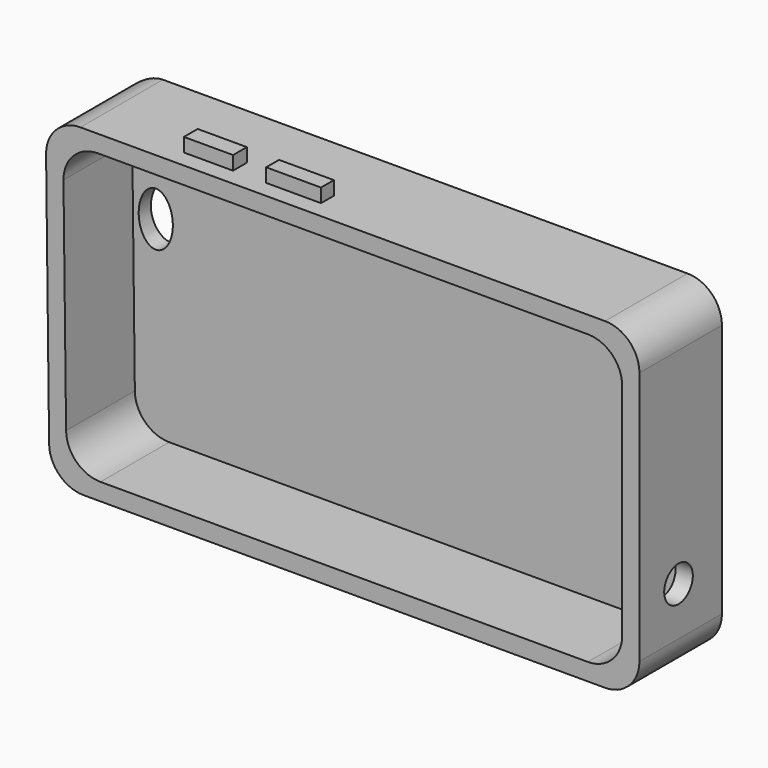
from build123d import *

# Parameters (mm, degrees)
F1_DEPTH    = 12.7
F2_T        = -2.54
F3_R        = 2.5336521523
F4_DEPTH    = 25.4
F5_W        = 12.6487519592
F5_H        = 3.011607565
F6_DEPTH    = 2.032
F7_T1_DEPTH = 51.1041796342
F7_T3_DEPTH = 73.1048124282
F7_T5_DEPTH = 50.4994199847
F7_T7_DEPTH = 50.8
F8_W        = 7.2596892715
F8_H        = 2.5458435994
F8_W_2      = 8.1038391218
F8_H_2      = 2.3770136759
F9_DEPTH    = 2.032
F11_DEPTH   = 5.334
F12_DEPTH   = 10.16
F13_R       = 5.08
F14_R       = 2.6429379381
F15_DEPTH   = 25.4


# Not quite as in the source:
# - a fillet or chamfer that OpenCascade refuses, or shapes differently, is made with other operations: its cross-section is extruded or revolved along the edge and cut away or added


with BuildPart() as f1:
    # F0 (on Front) → F1 (new body, symmetric)
    with BuildSketch(Plane.XZ):
        Polygon((37.1957607567, 37.33773157), (-50.5407974124, 37.33773157), (-49.9729253352, -10.3637007996), (37.1957607567, -10.3637007996), align=None)
    extrude(amount=F1_DEPTH, both=True)

    # F2
    f2_openings = [f1.faces().sort_by_distance(p)[0] for p in [
        (-6.530704, -12.7, 13.512828),
    ]]
    offset(amount=F2_T, openings=f2_openings)

    # F3 (on face) → F4 (cut)
    with BuildSketch(Plane.XZ.offset(-10.16)):
        with Locations((-44.7698123753, 30.0145167857)):
            Circle(F3_R)
    extrude(amount=-F4_DEPTH, mode=Mode.SUBTRACT)

    # F5 (on face) → F6 (join)
    with BuildSketch(Plane(origin=(0, 0, -10.3637007996), x_dir=(1, 0, 0), z_dir=(0, 0, -1))):
        with Locations((-34.2319430783, -6.4247637056)):
            Rectangle(F5_W, F5_H)
    extrude(amount=F6_DEPTH)

    # F7: fillet of radius 5.08 on 5 edges, made by hand

    # F7_s2 → F7_t1 (cut)
    with BuildSketch(Plane.XZ.offset(-25.5520898171)):
        with BuildLine():
            ThreePointArc((-50.4796015492, 32.19725989), (-49.0133806513, 35.8283900433), (-45.3999614856, 37.33773157))
            Line((-45.3999614856, 37.33773157), (-50.5407974124, 37.33773157))
            Line((-50.5407974124, 37.33773157), (-50.4796015492, 32.19725989))
        make_face()
    extrude(amount=F7_T1_DEPTH, mode=Mode.SUBTRACT)

    # F7_s4 → F7_t3 (cut)
    with BuildSketch(Plane(origin=(-0.602773104, 0, 50.6331295472), x_dir=(0, 1, 0), z_dir=(0.011903874, 0, -0.9999291464))):
        with BuildLine():
            ThreePointArc((12.7, -45.0127527613), (11.2121024484, -48.6048552097), (7.62, -50.0927527613))
            Line((7.62, -50.0927527613), (12.7, -50.0927527613))
            Line((12.7, -50.0927527613), (12.7, -45.0127527613))
        make_face()
    extrude(amount=F7_T3_DEPTH, mode=Mode.SUBTRACT)

    # F7_s6 → F7_t5 (cut)
    with BuildSketch(Plane.XZ.offset(-25.2497099923)):
        with BuildLine():
            ThreePointArc((-44.9530413382, -10.3637007996), (-48.5236998115, -8.8971199654), (-50.0326814019, -5.3441724797))
            Line((-50.0326814019, -5.3441724797), (-49.9729253352, -10.3637007996))
            Line((-49.9729253352, -10.3637007996), (-44.9530413382, -10.3637007996))
        make_face()
    extrude(amount=F7_T5_DEPTH, mode=Mode.SUBTRACT)

    # F7_s8 → F7_t7 (cut)
    with BuildSketch(Plane.XZ.offset(-25.4)):
        with BuildLine():
            ThreePointArc((32.1157607567, -10.3637007996), (35.7078632052, -8.8758032481), (37.1957607567, -5.2837007996))
            Line((37.1957607567, -5.2837007996), (37.1957607567, -10.3637007996))
            Line((37.1957607567, -10.3637007996), (32.1157607567, -10.3637007996))
        make_face()
        with BuildLine():
            ThreePointArc((37.1957607567, 32.25773157), (35.7078632052, 35.8498340184), (32.1157607567, 37.33773157))
            Line((32.1157607567, 37.33773157), (37.1957607567, 37.33773157))
            Line((37.1957607567, 37.33773157), (37.1957607567, 32.25773157))
        make_face()
    extrude(amount=F7_T7_DEPTH, mode=Mode.SUBTRACT)

    # F8 (on face) → F9 (join)
    with BuildSketch(Plane.XY.offset(37.33773157)):
        with Locations((-28.5155698657, 1.2729217997)):
            Rectangle(F8_W, F8_H)
        with Locations((-15.9377348609, 1.1885068379)):
            Rectangle(F8_W_2, F8_H_2)
    extrude(amount=F9_DEPTH)

    # F10 (on face) → F11 (cut)
    with BuildSketch(Plane.XZ.offset(-10.16)):
        with BuildLine():
            add(Edge.make_bspline(
                [(-44.4320701063, 24.525936693), (-48.8002594528, 24.525936693), (-46.6161647795, 18.5632575303), (-44.4320701063, 12.6005783677), (-42.247975433, 18.5632575303), (-40.0638807598, 24.525936693), (-44.4320701063, 24.525936693)],
                knots=[0, 0, 0, 2.0943951024, 2.0943951024, 4.1887902048, 4.1887902048, 6.2831853072, 6.2831853072, 6.2831853072], degree=2, weights=[1, 0.5, 1, 0.5, 1, 0.5, 1]))
        make_face()
    extrude(amount=-F11_DEPTH, mode=Mode.SUBTRACT)

    # F12 (cut): a face of the model
    f12_faces = [f1.faces().sort_by_distance(p)[0] for p in [
        (-48.3034140755, -12.7, 35.1268251117),
    ]]
    extrude(f12_faces, amount=-F12_DEPTH, mode=Mode.SUBTRACT)

    # F13
    f13_edges = [f1.edges().sort_by_distance(p)[0] for p in [
        (-47.462983, 3.81, -7.823701),
        (-47.970379, 3.81, 34.797732),
        (34.655761, 3.81, -7.823701),
        (34.655761, 3.81, 34.797732),
    ]]
    fillet(f13_edges, radius=F13_R)

    # F14 (on face) → F15 (cut)
    with BuildSketch(Plane.YZ.offset(37.1957607567)):
        with Locations((4.6823634766, 1.8731907476)):
            Circle(F14_R)
    extrude(amount=-F15_DEPTH, mode=Mode.SUBTRACT)


solid = f1.part
